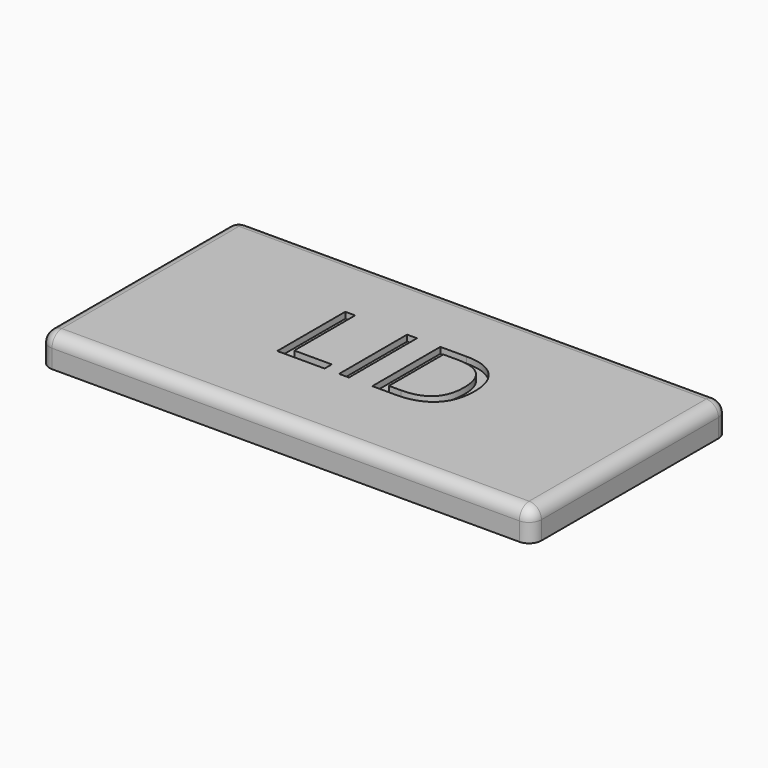
from build123d import *

# Parameters (mm, degrees)
F0_W         = 101.6
F0_H         = 50.8
F1_DEPTH     = 6.35
F2_T         = -2.54
F3_R         = 2.54
F4_TEXT_SIZE = 24.6073476123
F5_DEPTH     = 1.27


# Not quite as in the source:
# - Text() gives the source's letters only with a copy of the font that has no kerning and outlines rounded to 1/6400 em; it was checked with that copy


with BuildPart() as f1:
    # F0 (on Top) → F1 (new body)
    with BuildSketch(Plane.XY):
        with Locations((-19.0189632024, 0.9936690331)):
            Rectangle(F0_W, F0_H)
    extrude(amount=F1_DEPTH)

    # F2
    f2_openings = [f1.faces().sort_by_distance(p)[0] for p in [
        (-19.018963, 0.993669, 0),
    ]]
    offset(amount=F2_T, openings=f2_openings)

    # F3
    f3_edges = [f1.edges().sort_by_distance(p)[0] for p in [
        (-19.018963, 26.393669, 6.35),
        (-69.818963, 0.993669, 6.35),
        (-19.018963, -24.406331, 6.35),
        (31.781037, 0.993669, 6.35),
        (-69.818963, -24.406331, 3.175),
        (31.781037, -24.406331, 3.175),
        (31.781037, 26.393669, 3.175),
        (-69.818963, 26.393669, 3.175),
    ]]
    fillet(f3_edges, radius=F3_R)

    # F4 (on face) → F5 (cut)
    with BuildSketch(Plane.XY.offset(6.35)):
        with Locations((-37.664621439, -6.2858246965)):
            Text('LID', F4_TEXT_SIZE, font='Open Sans', text_align=(TextAlign.LEFT, TextAlign.BOTTOM))
    extrude(amount=-F5_DEPTH, mode=Mode.SUBTRACT)


solid = f1.part
